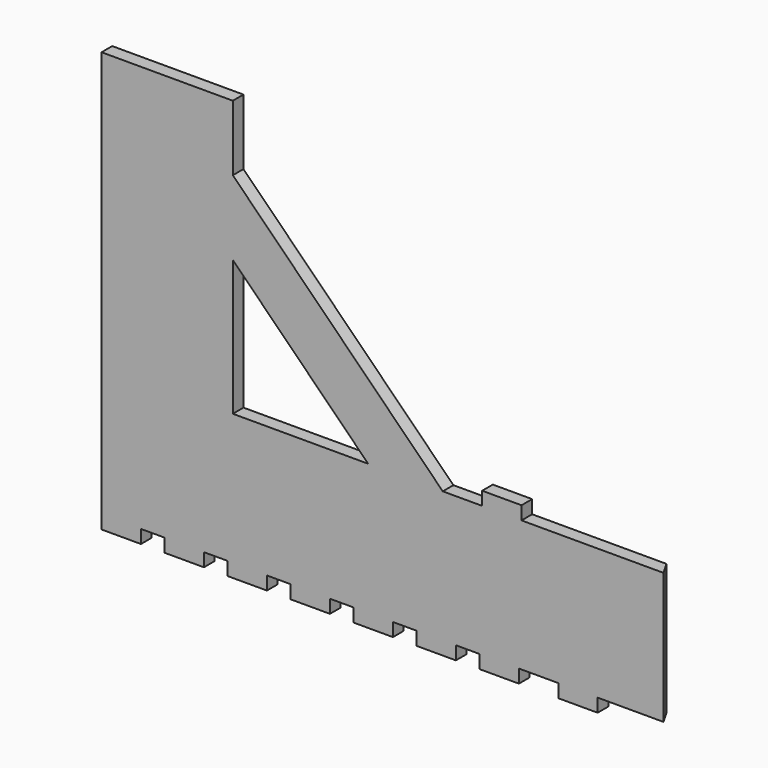
from build123d import *

# Parameters (mm, degrees)
F0_W     = 15
F0_H     = 5.08
F1_DEPTH = 5.08
F2_DEPTH = 25
F4_DEPTH = 58
F5_W     = 15
F5_H     = 5.08
F6_DEPTH = 5.08
F7_W     = 15
F7_H     = 5.08
F8_DEPTH = 5.08


# Not quite as in the source:
# - a feature names something its author has since deleted; it is built from what else it names


with BuildPart() as f1:
    # F0 (on Front) → F1 (new body)
    with BuildSketch(Plane.XZ):
        Polygon((-87.5, 0), (-32.419, 0), (-32.419, 50), (-116.5, 50), (-144.9023774395, 50), (-196.5, 50), (-196.5, 101.5976225605), (-196.5, 130), (-246.5, 130), (-246.5, 0), (-231.5, 0), (-222.5, 0), (-207.5, 0), (-198.5, 0), (-183.5, 0), (-174.5, 0), (-159.5, 0), (-150.5, 0), (-135.5, 0), (-126.5, 0), (-111.5, 0), (-102.5, 0), align=None)
        with Locations((-95, -2.54)):
            Rectangle(F0_W, F0_H)
        Polygon((-144.9023774395, 50), (-116.5, 50), (-196.5, 130), (-196.5, 101.5976225605), align=None)
        with Locations((-119, -2.54)):
            Rectangle(F0_W, F0_H)
        with Locations((-143, -2.54)):
            Rectangle(F0_W, F0_H)
        with Locations((-239, -2.54)):
            Rectangle(F0_W, F0_H)
        with Locations((-167, -2.54)):
            Rectangle(F0_W, F0_H)
        with Locations((-215, -2.54)):
            Rectangle(F0_W, F0_H)
        with Locations((-191, -2.54)):
            Rectangle(F0_W, F0_H)
    extrude(amount=F1_DEPTH)

    # F2 (add): a face of the model
    f2_faces = [f1.faces().sort_by_distance(p)[0] for p in [
        (-221.5, -2.54, 130),
    ]]
    extrude(f2_faces, amount=F2_DEPTH)

    # F3 (on face) → F4 (cut)
    with BuildSketch(Plane(origin=(0, 0, 0), x_dir=(1, 0, 0), z_dir=(0, 0, -1))):
        Polygon((-32.419, 0), (-32.419, 5.08), (-35.3519393675, 0), align=None)
    extrude(amount=-F4_DEPTH, mode=Mode.SUBTRACT)

    # F5 (on face) → F6 (join)
    with BuildSketch(Plane(origin=(0, 0, 0), x_dir=(1, 0, 0), z_dir=(0, 0, -1))):
        with Locations((-65, 2.54)):
            Rectangle(F5_W, F5_H)
    extrude(amount=F6_DEPTH)

    # F7 (on face) → F8 (join)
    with BuildSketch(Plane.XY.offset(50)):
        with Locations((-94, -2.54)):
            Rectangle(F7_W, F7_H)
    extrude(amount=F8_DEPTH)


solid = f1.part
